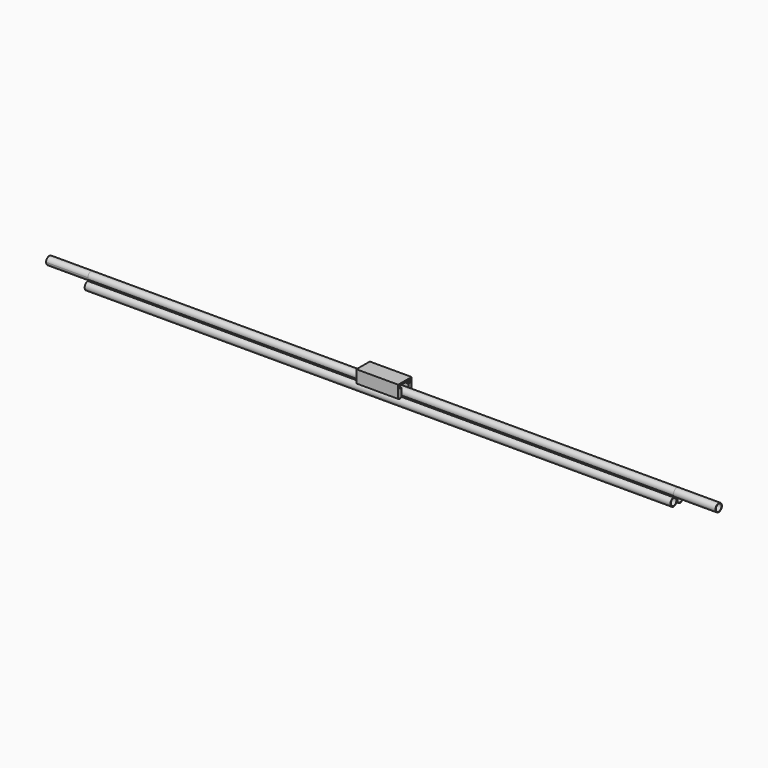
from build123d import *
from build123d import SkipClean  # not in build123d's __all__

# Parameters (mm, degrees)
F0_R      = 20.65
F1_DEPTH  = 4000
F2_W      = 120.345171541
F2_H      = 96.7681743205
F2_R      = 24.15
F3_DEPTH  = 250
F4_W      = 149.252615869
F4_H      = 108.2491464913
F4_R      = 24.15
F5_DEPTH  = 250
F9_DEPTH  = 125
F10_W     = 50
F10_H     = 15
F11_DEPTH = 50
F13_DEPTH = 50
F15_DEPTH = 50


# Not quite as in the source:
# - after a boolean that leaves OpenCascade's solid faulty, fix() repairs it


with BuildPart() as f1:
    # F0 (on Right) → F1 (new body)
    with BuildSketch(Plane.YZ):
        with BuildLine():
            Line((-20.8711227654, 12.0001549593), (-24.0634869254, 6.4708180379))
            ThreePointArc((-24.0634869254, 6.4708180379), (-45.0645135014, -29.7540270028), (-3.19236416, -29.6790270028))
            Line((-3.19236416, -29.6790270028), (3.19236416, -29.6790270028))
            ThreePointArc((3.19236416, -29.6790270028), (45.0645135014, -29.7540270028), (24.0634869254, 6.4708180379))
            Line((24.0634869254, 6.4708180379), (20.8711227654, 12.0001549593))
            ThreePointArc((20.8711227654, 12.0001549593), (0, 48.3), (-20.8711227654, 12.0001549593))
        make_face()
        with Locations((-24.15, -17.6790270028)):
            Circle(F0_R, mode=Mode.SUBTRACT)
        with BuildLine():
            ThreePointArc((-12.075, 3.2354864986), (-6.2922525862, 0.8341243486), (-0.0865130746, 0.0001549593))
            ThreePointArc((-0.0865130746, 0.0001549593), (0, 0), (0.0865130746, 0.0001549593))
            ThreePointArc((0.0865130746, 0.0001549593), (6.2922525862, 0.8341243486), (12.075, 3.2354864986))
            ThreePointArc((12.075, 3.2354864986), (7.1039856675, -0.5718385904), (3.2788772346, -5.5291819621))
            ThreePointArc((3.2788772346, -5.5291819621), (3.2354864986, -5.6040270028), (3.19236416, -5.6790270028))
            ThreePointArc((3.19236416, -5.6790270028), (0.8117330813, -11.4703397637), (0, -17.6790270028))
            ThreePointArc((0, -17.6790270028), (-0.8117330813, -11.4703397637), (-3.19236416, -5.6790270028))
            ThreePointArc((-3.19236416, -5.6790270028), (-3.2354864986, -5.6040270028), (-3.2788772346, -5.5291819621))
            ThreePointArc((-3.2788772346, -5.5291819621), (-7.1039856675, -0.5718385904), (-12.075, 3.2354864986))
        make_face(mode=Mode.SUBTRACT)
        with Locations((24.15, -17.6790270028)):
            Circle(F0_R, mode=Mode.SUBTRACT)
        with Locations((0, 24.15)):
            Circle(F0_R, mode=Mode.SUBTRACT)
    extrude(amount=-F1_DEPTH)

    # F2 (on face) → F3 (cut)
    with BuildSketch(Plane(origin=(-4000, 0, 0), x_dir=(0, -1, 0), z_dir=(-1, 0, 0))):
        with Locations((-0.3221537918, 0.9117070585)):
            Rectangle(F2_W, F2_H)
        with Locations((0, 24.15)):
            Circle(F2_R, mode=Mode.SUBTRACT)
    with SkipClean():  # cleaning this boolean's faces spoils the solid; the shape is the same uncleaned
        extrude(amount=-F3_DEPTH, mode=Mode.SUBTRACT)

    # F4 (on face) → F5 (cut)
    with BuildSketch(Plane.YZ):
        with Locations((-4.9993358552, 3.1689684838)):
            Rectangle(F4_W, F4_H)
        with Locations((0, 24.15)):
            Circle(F4_R, mode=Mode.SUBTRACT)
    extrude(amount=-F5_DEPTH, mode=Mode.SUBTRACT)

    add(f1.part.fix(), mode=Mode.REPLACE)



with BuildPart() as f9:
    # F8 (on mid) → F9 (new body, symmetric)
    with BuildSketch(Plane(origin=(-2000, 0, 0), x_dir=(0, -1, 0), z_dir=(-1, 0, 0))):
        Polygon((50, 6.4708180379), (50, 81.4708180379), (-50, 81.4708180379), (-50, 6.4708180379), (-40, 6.4708180379), (-40, 71.4708180379), (40, 71.4708180379), (40, 6.4708180379), align=None)
    extrude(amount=F9_DEPTH, both=True)

    # F10 (on face) → F11 (join)
    with BuildSketch(Plane(origin=(0, 0, 6.4708180379), x_dir=(1, 0, 0), z_dir=(0, 0, -1))):
        with Locations((-2100, 32.5)):
            Rectangle(F10_W, F10_H)
        with Locations((-1900, 32.5)):
            Rectangle(F10_W, F10_H)
        with Locations((-1900, -32.5)):
            Rectangle(F10_W, F10_H)
        with Locations((-2100, -32.5)):
            Rectangle(F10_W, F10_H)
    extrude(amount=-F11_DEPTH)


with BuildPart() as f1_1:
    add(f1.part, clean=False)

    add(f9.part)  # F13 merges F9
    # F12 (on face) → F13 (join, through all)
    with BuildSketch(Plane(origin=(-2125, 0, 0), x_dir=(0, -1, 0), z_dir=(-1, 0, 0))):
        with BuildLine():
            Line((40, 6.4708180379), (25, 6.4708180379))
            Line((25, 6.4708180379), (25, 2.9534716341))
            ThreePointArc((25, 2.9534716341), (33.282271785, 0.8418831272), (40, -4.4427133166))
            Line((40, -4.4427133166), (40, 6.4708180379))
        make_face()
        with BuildLine():
            Line((-25, 6.4708180379), (-40, 6.4708180379))
            Line((-40, 6.4708180379), (-40, -4.4427133166))
            ThreePointArc((-40, -4.4427133166), (-33.282271785, 0.8418831272), (-25, 2.9534716341))
            Line((-25, 2.9534716341), (-25, 6.4708180379))
        make_face()
    extrude(amount=-F13_DEPTH)

    # F14 (on face) → F15 (join, through all)
    with BuildSketch(Plane.YZ.offset(-1875)):
        with BuildLine():
            Line((40, -4.4427133166), (40, 6.4708180379))
            Line((40, 6.4708180379), (25, 6.4708180379))
            Line((25, 6.4708180379), (25, 2.9534716341))
            ThreePointArc((25, 2.9534716341), (33.282271785, 0.8418831272), (40, -4.4427133166))
        make_face()
        with BuildLine():
            Line((-25, 6.4708180379), (-40, 6.4708180379))
            Line((-40, 6.4708180379), (-40, -4.4427133166))
            ThreePointArc((-40, -4.4427133166), (-33.282271785, 0.8418831272), (-25, 2.9534716341))
            Line((-25, 2.9534716341), (-25, 6.4708180379))
        make_face()
    extrude(amount=-F15_DEPTH)


solid = f1_1.part
